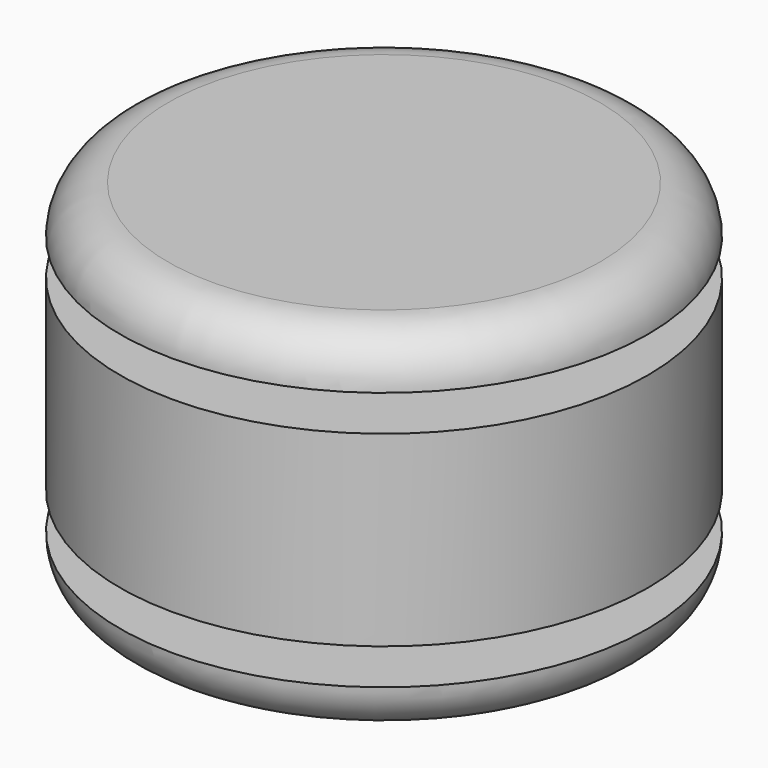
from build123d import *
from build123d import SkipClean  # not in build123d's __all__

# Parameters (mm, degrees)
F0_R      = 5.4
F1_DEPTH  = 1.5
F2_R      = 8.4
F2_R_2    = 6.4
F3_DEPTH  = 4.8
F4_R      = 11
F4_R_2    = 8.4
F5_DEPTH  = 7.8
F6_R      = 11
F6_R_2    = 5.4
F7_DEPTH  = 1.5
F8_R      = 3.175
F9_DEPTH  = 4.8
F10_R     = 4.175
F11_DEPTH = 3
F12_R     = 11
F13_DEPTH = 2
F14_R     = 1.95
F15_DEPTH = 7.4
F16_R     = 1.99999
F17_R     = 4.175
F18_DEPTH = 3
F19_R     = 11
F20_DEPTH = 2
F21_R     = 1.95
F22_DEPTH = 2.6
F23_R     = 1.99999


# Not quite as in the source:
# - a fillet or chamfer is up to 0.001 mm smaller than in the source, because OpenCascade refuses the exact size


with BuildPart() as f1:
    # F0 (on Top) → F1 (new body)
    with BuildSketch(Plane.XY):
        with BuildLine():
            ThreePointArc((2.5007633588, 8.0191135809), (0, 8.4), (-2.5007633588, 8.0191135809))
            ThreePointArc((-2.5007633588, 8.0191135809), (-7.2746133918, 4.2), (-8.1951377563, -1.8438321929))
            ThreePointArc((-8.1951377563, -1.8438321929), (-7.2746133918, -4.2), (-5.6943743975, -6.175281388))
            ThreePointArc((-5.6943743975, -6.175281388), (0, -8.4), (5.6943743975, -6.175281388))
            ThreePointArc((5.6943743975, -6.175281388), (7.2746133918, -4.2), (8.1951377563, -1.8438321929))
            ThreePointArc((8.1951377563, -1.8438321929), (7.2746133918, 4.2), (2.5007633588, 8.0191135809))
        make_face()
        Circle(F0_R, mode=Mode.SUBTRACT)
    extrude(amount=-F1_DEPTH)

    # F2 (on face) → F3 (join)
    with BuildSketch(Plane.XY):
        Circle(F2_R)
        Circle(F2_R_2, mode=Mode.SUBTRACT)
    with SkipClean():  # cleaning this boolean's faces spoils the solid; the shape is the same uncleaned
        extrude(amount=F3_DEPTH)



with BuildPart() as f5:
    # F4 (on face) → F5 (new body)
    with BuildSketch(Plane(origin=(0, 0, -1.5), x_dir=(1, 0, 0), z_dir=(0, 0, -1))):
        Circle(F4_R)
        Circle(F4_R_2, mode=Mode.SUBTRACT)
    extrude(amount=-F5_DEPTH)


with BuildPart() as f1_1:
    add(f1.part, clean=False)

    add(f5.part)  # F7 merges F5
    # F6 (on face) → F7 (join)
    with BuildSketch(Plane.XY.offset(6.3)):
        Circle(F6_R)
        Circle(F6_R_2, mode=Mode.SUBTRACT)
    extrude(amount=-F7_DEPTH)


with BuildPart() as f9:
    # F8 (on face) → F9 (new body)
    with BuildSketch(Plane.XY):
        Circle(F8_R)
    extrude(amount=F9_DEPTH)

    # F10 (on face) → F11 (join, through all)
    with BuildSketch(Plane(origin=(0, 0, 0), x_dir=(1, 0, 0), z_dir=(0, 0, -1))):
        Circle(F10_R)
    extrude(amount=F11_DEPTH)

    # F12 (on face) → F13 (join)
    with BuildSketch(Plane(origin=(0, 0, -3), x_dir=(1, 0, 0), z_dir=(0, 0, -1))):
        Circle(F12_R)
    extrude(amount=F13_DEPTH)

    # F14 (on face) → F15 (cut)
    with BuildSketch(Plane.XY.offset(4.8)):
        Circle(F14_R)
    extrude(amount=-F15_DEPTH, mode=Mode.SUBTRACT)

    # F16 (radius 2 in the source; OpenCascade refuses exactly that, so slightly less here)
    f16_edges = [f9.edges().sort_by_distance(p)[0] for p in [
        (-4.175, 0, -3),
        (-11, 0, -5),
    ]]
    fillet(f16_edges, radius=F16_R)


with BuildPart() as f18:
    # F17 (on face) → F18 (new body, through all)
    with BuildSketch(Plane.XY.offset(4.8)):
        Circle(F17_R)
    extrude(amount=F18_DEPTH)

    # F19 (on face) → F20 (join)
    with BuildSketch(Plane.XY.offset(7.8)):
        Circle(F19_R)
    extrude(amount=F20_DEPTH)

    # F21 (on face) → F22 (cut)
    with BuildSketch(Plane(origin=(0, 0, 4.8), x_dir=(1, 0, 0), z_dir=(0, 0, -1))):
        Circle(F21_R)
    extrude(amount=-F22_DEPTH, mode=Mode.SUBTRACT)

    # F23 (radius 2 in the source; OpenCascade refuses exactly that, so slightly less here)
    f23_edges = [f18.edges().sort_by_distance(p)[0] for p in [
        (-11, 0, 9.8),
        (-4.175, 0, 7.8),
    ]]
    fillet(f23_edges, radius=F23_R)


solid = Compound([f1_1.part, f9.part, f18.part])
